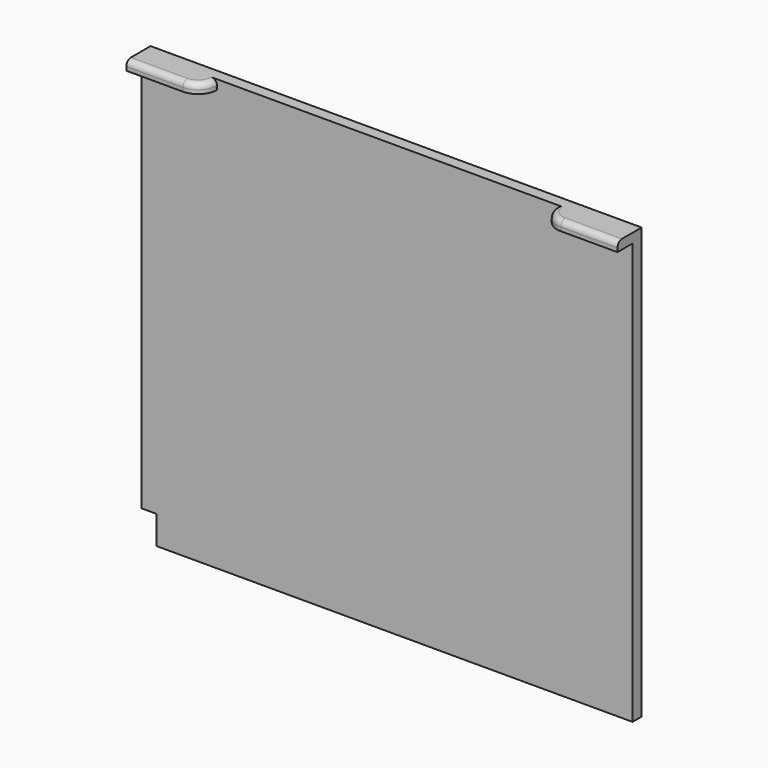
from build123d import *

# Parameters (mm, degrees)
F0_W     = 130
F0_H     = 114
F1_DEPTH = 3
F2_W     = 20
F2_H     = 2.5
F3_DEPTH = 5
F4_R     = 4.99999
F5_R     = 1.5
F6_W     = 4
F6_H     = 7.5
F7_DEPTH = 25


# Not quite as in the source:
# - a fillet or chamfer is up to 0.001 mm smaller than in the source, because OpenCascade refuses the exact size


with BuildPart() as f1:
    # F0 (on Front) → F1 (new body)
    with BuildSketch(Plane.XZ):
        with Locations((65, 57)):
            Rectangle(F0_W, F0_H)
    extrude(amount=F1_DEPTH)

    # F2 (on face) → F3 (join)
    with BuildSketch(Plane.XZ.offset(3)):
        with Locations((10, 112.75)):
            Rectangle(F2_W, F2_H)
        with Locations((120, 112.75)):
            Rectangle(F2_W, F2_H)
    extrude(amount=F3_DEPTH)

    # F4 (radius 5 in the source; OpenCascade refuses exactly that, so slightly less here)
    f4_edges = [f1.edges().sort_by_distance(p)[0] for p in [
        (20, -8, 112.75),
        (110, -8, 112.75),
    ]]
    fillet(f4_edges, radius=F4_R)

    # F5
    f5_edges = [f1.edges().sort_by_distance(p)[0] for p in [
        (7.500005, -8, 114),
        (122.499995, -8, 114),
    ]]
    fillet(f5_edges, radius=F5_R)

    # F6 (on face) → F7 (cut)
    with BuildSketch(Plane(origin=(0, 0, 0), x_dir=(-1, 0, 0), z_dir=(0, 1, 0))):
        with Locations((-2, 3.75)):
            Rectangle(F6_W, F6_H)
    extrude(amount=-F7_DEPTH, mode=Mode.SUBTRACT)


solid = f1.part
